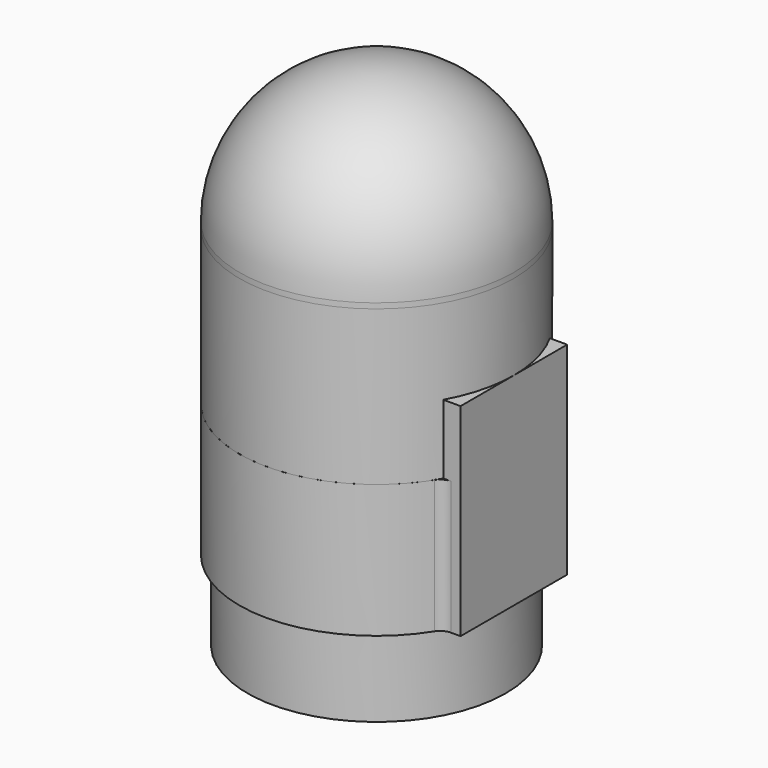
from build123d import *

# Parameters (mm, degrees)
F3_W     = 50
F3_H     = 76
F4_DEPTH = 10.2
F11_R    = 5


with BuildPart() as f1:
    # F0 (on Front) → F1 (revolve)
    with BuildSketch(Plane.XZ):
        Polygon((46.5, 32), (46.5, 0), (48.5, 0), (48.5, 30), (51.5, 30), (51.5, 80), (50.5, 80), (50.5, 82), (49.5, 82), (49.5, 37.1961524227), align=None)
    revolve(axis=Axis((0, 0, 67.2105439007), (0, 0, -1)))

    # F3 (on plane+point) → F4 (join)
    with BuildSketch(Plane.YZ.offset(51.5)):
        with Locations((0, 68)):
            Rectangle(F3_W, F3_H)
    extrude(amount=-F4_DEPTH)


with BuildPart() as f6:
    # F5 (on Front) → F6 (revolve)
    with BuildSketch(Plane.XZ):
        Polygon((49.5, 140), (49.5, 82), (50.5, 82), (50.5, 80), (51.5, 80), (51.5, 140), align=None)
    revolve(axis=Axis((0, 0, 67.2105439007), (0, 0, -1)))


with BuildPart() as f8:
    # F7 (on Front) → F8 (revolve)
    with BuildSketch(Plane.XZ):
        with BuildLine():
            Line((50.5, 138), (51.5, 138))
            Line((51.5, 138), (51.5, 140))
            ThreePointArc((51.5, 140), (36.4159992311, 176.4159992311), (0, 191.5))
            Line((0, 191.5), (0, 189.5))
            ThreePointArc((0, 189.5), (35.0017856687, 175.0017856687), (49.5, 140))
            Line((49.5, 140), (50.5, 140))
            Line((50.5, 140), (50.5, 138))
        make_face()
    revolve(axis=Axis((0, 0, 67.2105439007), (0, 0, -1)))


with BuildPart() as f6_1:
    add(f6.part)

    # F9: cut F8
    add(f8.part, mode=Mode.SUBTRACT)

    # F10: cut F1
    add(f1.part, mode=Mode.SUBTRACT)


with BuildPart() as f1_1:
    add(f1.part)

    # F11
    f11_edges = [f1_1.edges().sort_by_distance(p)[0] for p in [
        (45.024993, -25, 55),
        (45.024993, 25, 55),
    ]]
    fillet(f11_edges, radius=F11_R)


solid = Compound([f8.part, f6_1.part, f1_1.part])
